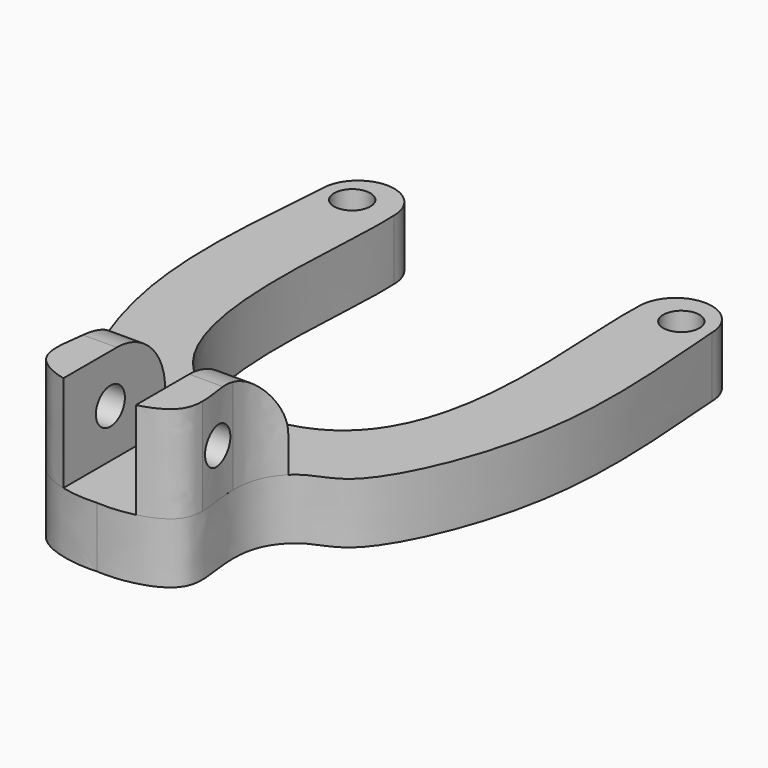
from build123d import *

# Parameters (mm, degrees)
F0_R     = 1.5
F1_DEPTH = 5
F3_DEPTH = 8
F4_R     = 5
F5_R     = 5
F6_R     = 1.5
F7_DEPTH = 25
F8_DEPTH = 25


with BuildPart() as f1:
    # F0 (on Top) → F1 (new body)
    with BuildSketch(Plane.XY):
        with BuildLine():
            add(Edge.make_bspline(
                [(16.1482299072, 51.6973561981), (16.5899840055, 45.719780335), (17.7869330039, 34.5645654052), (11.8866558986, 20.6767048109), (8.0186883827, 20.0792477956), (5.7487297616, 17.5830961458), (5.6074196408, 13.9410727562), (6.7948821633, 9.1867459415), (2.0567567076, 8.1085397531), (0, 8.2666967064)],
                knots=[0, 0, 0, 0, 0.2391514832, 0.4458745748, 0.5478772622, 0.6443235313, 0.7519815522, 0.8637763281, 1, 1, 1, 1], degree=3))
            ThreePointArc((16.1482299191, 51.6973561981), (15.239687494, 53.8481247147), (13.0643597776, 54.6961836021))
            ThreePointArc((13.0643597776, 54.6961836021), (10.9974614024, 53.788813773), (10.1482299191, 51.6973561981))
            add(Edge.make_bspline(
                [(10.1482299191, 51.6973561981), (9.727734266, 44.379245697), (14.0333045274, 24.2629591376), (0, 24.1981324146)],
                knots=[0, 0, 0, 0, 29.3120091291, 29.3120091291, 29.3120091291, 29.3120091291], degree=3))
            add(Edge.make_bspline(
                [(-10.1482299072, 51.6973561981), (-9.7277342541, 44.379245697), (-14.0333045274, 24.2629591376), (0, 24.1981324146)],
                knots=[0, 0, 0, 0, 29.3120091249, 29.3120091249, 29.3120091249, 29.3120091249], degree=3))
            ThreePointArc((-10.1482299072, 51.6973561981), (-10.9974613905, 53.788813773), (-13.0643597657, 54.6961836021))
            ThreePointArc((-13.0643597657, 54.6961836021), (-15.2396874821, 53.8481247147), (-16.1482299072, 51.6973561981))
            add(Edge.make_bspline(
                [(-16.1482299072, 51.6973561981), (-16.5899840055, 45.719780335), (-17.7869330039, 34.5645654052), (-11.8866558986, 20.6767048109), (-8.0186883827, 20.0792477956), (-5.7487297616, 17.5830961458), (-5.6074196408, 13.9410727562), (-6.7948821633, 9.1867459415), (-2.0567567076, 8.1085397531), (0, 8.2666967064)],
                knots=[0, 0, 0, 0, 0.2391514832, 0.4458745748, 0.5478772622, 0.6443235313, 0.7519815522, 0.8637763281, 1, 1, 1, 1], degree=3))
        make_face()
        with Locations((0, 21.2669761981)):
            Circle(F0_R, mode=Mode.SUBTRACT)
        with Locations((-13.6254811949, 51.6973561981)):
            Circle(F0_R, mode=Mode.SUBTRACT)
        with Locations((13.6254812068, 51.6973561981)):
            Circle(F0_R, mode=Mode.SUBTRACT)
    extrude(amount=F1_DEPTH)

    # F2 (on face) → F3 (join)
    with BuildSketch(Plane.XY.offset(5)):
        with BuildLine():
            add(Edge.make_bspline(
                [(7.1994148887, 19.0504361046), (6.7623605443, 18.624380519), (5.9486349037, 17.4664030432), (5.7310142999, 16.0197452548), (5.7312992126, 15.1677248801)],
                knots=[0.5847071296, 0.5847071296, 0.5847071296, 0.5847071296, 0.6443235313, 0.7168445185, 0.7168445185, 0.7168445185, 0.7168445185], degree=3))
            Line((7.1994148887, 19.0504361046), (3, 19.0504361046))
            Line((3, 19.0504361046), (3, 8.525359011))
            add(Edge.make_bspline(
                [(6.0411689582, 11.6423631069), (6.0408139506, 11.0240402402), (5.7782021371, 9.6331058885), (4.1142488605, 8.8053747205), (3, 8.525359011)],
                knots=[0.8121984251, 0.8121984251, 0.8121984251, 0.8121984251, 0.8637763281, 0.9366436123, 0.9366436123, 0.9366436123, 0.9366436123], degree=3))
            add(Edge.make_bspline(
                [(5.7312992126, 15.1677248801), (5.7311604373, 14.7530215017), (5.807523228, 13.5958597841), (6.0407562033, 12.3625435353), (6.0411689582, 11.6423631069)],
                knots=[0.7166720019, 0.7166720019, 0.7166720019, 0.7166720019, 0.7519815522, 0.8120294204, 0.8120294204, 0.8120294204, 0.8120294204], degree=3))
        make_face()
        with BuildLine():
            Line((-3, 8.525359011), (-3, 19.0504361046))
            Line((-3, 19.0504361046), (-7.1994148887, 19.0504361046))
            add(Edge.make_bspline(
                [(-7.1994148887, 19.0504361046), (-6.7623605443, 18.624380519), (-5.9486349037, 17.4664030432), (-5.7310142999, 16.0197452548), (-5.7312992126, 15.1677248801)],
                knots=[0.5847071296, 0.5847071296, 0.5847071296, 0.5847071296, 0.6443235313, 0.7168445185, 0.7168445185, 0.7168445185, 0.7168445185], degree=3))
            add(Edge.make_bspline(
                [(-5.7312992126, 15.1677248801), (-5.7311604373, 14.7530215017), (-5.807523228, 13.5958597841), (-6.0407562033, 12.3625435353), (-6.0411689582, 11.6423631069)],
                knots=[0.7166720019, 0.7166720019, 0.7166720019, 0.7166720019, 0.7519815522, 0.8120294204, 0.8120294204, 0.8120294204, 0.8120294204], degree=3))
            add(Edge.make_bspline(
                [(-6.0411689582, 11.6423631069), (-6.0408139506, 11.0240402402), (-5.7782021371, 9.6331058885), (-4.1142488605, 8.8053747205), (-3, 8.525359011)],
                knots=[0.8121984251, 0.8121984251, 0.8121984251, 0.8121984251, 0.8637763281, 0.9366436123, 0.9366436123, 0.9366436123, 0.9366436123], degree=3))
        make_face()
    extrude(amount=F3_DEPTH)

    # F4
    f4_edges = [f1.edges().sort_by_distance(p)[0] for p in [
        (-5.099707, 19.050436, 13),
    ]]
    fillet(f4_edges, radius=F4_R)

    # F5
    f5_edges = [f1.edges().sort_by_distance(p)[0] for p in [
        (5.099707, 19.050436, 13),
    ]]
    fillet(f5_edges, radius=F5_R)

    # F6 (on Right) → F7 (cut)
    with BuildSketch(Plane.YZ):
        with Locations((13.3909519742, 9)):
            Circle(F6_R)
    extrude(amount=-F7_DEPTH, mode=Mode.SUBTRACT)

    # F6 (on Right) → F8 (cut)
    with BuildSketch(Plane.YZ):
        with Locations((13.3909519742, 9)):
            Circle(F6_R)
    extrude(amount=F8_DEPTH, mode=Mode.SUBTRACT)


solid = f1.part
